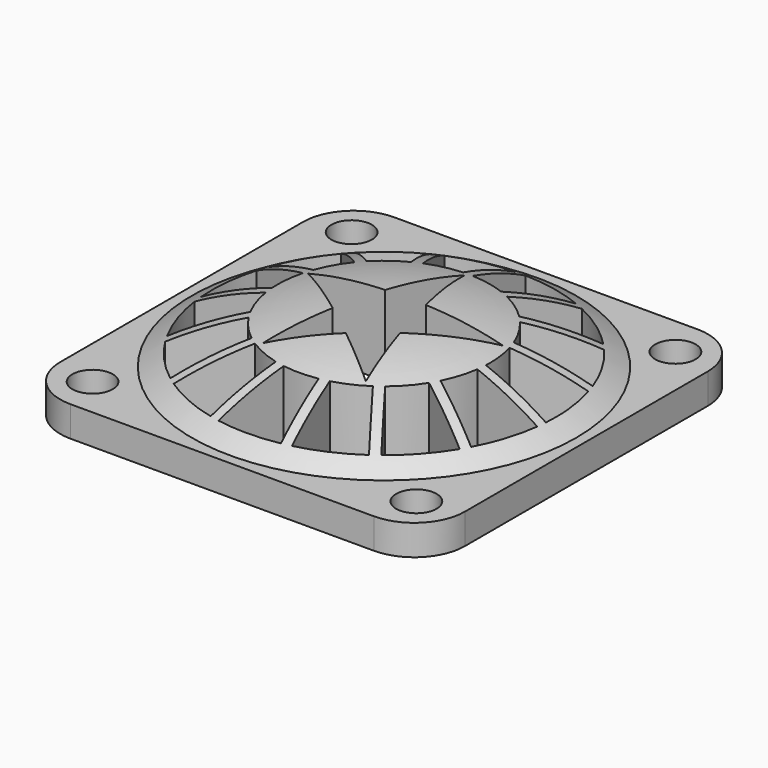
from build123d import *

# Parameters (mm, degrees)
F0_W      = 40
F0_H      = 40
F1_DEPTH  = 3
F2_R      = 2
F3_DEPTH  = 25
F4_R      = 19
F5_DEPTH  = 5
F8_DEPTH  = 25
F10_DEPTH = 25
F11_R     = 5
F12_R     = 5
F13_R     = 5
F14_R     = 5


# Not quite as in the source:
# - a fillet or chamfer that OpenCascade refuses, or shapes differently, is made with other operations: its cross-section is extruded or revolved along the edge and cut away or added


with BuildPart() as f1:
    # F0 (on Top) → F1 (new body)
    with BuildSketch(Plane.XY):
        with Locations((20, 20)):
            Rectangle(F0_W, F0_H)
    extrude(amount=F1_DEPTH)

    # F2 (on face) → F3 (cut)
    with BuildSketch(Plane.XY.offset(3)):
        with Locations((4, 36)):
            Circle(F2_R)
        with Locations((36, 36)):
            Circle(F2_R)
        with Locations((36, 4)):
            Circle(F2_R)
        with Locations((4, 4)):
            Circle(F2_R)
    extrude(amount=-F3_DEPTH, mode=Mode.SUBTRACT)

    # F4 (on face) → F5 (join)
    with BuildSketch(Plane.XY.offset(3)):
        with Locations((20, 20)):
            Circle(F4_R)
    extrude(amount=F5_DEPTH)

    # F6: fillet of radius 33 on 1 edges, made by hand

    # F6_s1 → F6_t2 (revolve, cut)
    with BuildSketch(Plane.XZ.offset(-20)):
        with BuildLine():
            ThreePointArc((39, 3), (30.6187018657, 6.7253841584), (21.5357508034, 8))
            Line((21.5357508034, 8), (21.5357508034, 8.66))
            Line((21.5357508034, 8.66), (39, 8.66))
            Line((39, 8.66), (39.66, 8))
            ThreePointArc((39.66, 8), (39.66, 5.5), (39.3492849839, 3.56))
            Line((39.3492849839, 3.56), (39, 3))
        make_face()
    revolve(axis=Axis((20, 20, 8), (0, 0, 1)), mode=Mode.SUBTRACT)

    # F7 (on face) → F8 (cut)
    with BuildSketch(Plane.XY.offset(8)):
        Polygon((22.0111904992, 22.6488580818), (20, 30), (17.9888095008, 22.6488580818), (10.3572021248, 22.6488580818), (16.6694497764, 17.8264404242), (14.9092685387, 11.3927673908), (20, 15.2819736836), (25.0907314613, 11.3927673908), (23.3305502236, 17.8264404242), (29.6427978752, 22.6488580818), align=None)
    extrude(amount=-F8_DEPTH, mode=Mode.SUBTRACT)

    # F9 (on face) → F10 (cut)
    with BuildSketch(Plane(origin=(0, 0, 0), x_dir=(1, 0, 0), z_dir=(0, 0, -1))):
        with BuildLine():
            ThreePointArc((23.7333544181, -29.8138710399), (22.0791153795, -30.2920979027), (20.3689578921, -30.4935156203))
            Line((20.3689578921, -30.4935156203), (20.3689578921, -36.995995707))
            ThreePointArc((20.3689578921, -36.995995707), (23.4306499348, -36.6502444734), (26.3796468832, -35.757541231))
            Line((26.3796468832, -35.757541231), (23.7333544181, -29.8138710399))
        make_face()
        with BuildLine():
            ThreePointArc((13.4241655667, -35.6766833707), (16.3617901212, -36.6061262454), (19.4189280081, -36.9900663724))
            Line((19.4189280081, -36.9900663724), (19.4189280081, -30.4839093539))
            ThreePointArc((19.4189280081, -30.4839093539), (17.7131930598, -30.2479516987), (16.0689624889, -29.7363722241))
            Line((16.0689624889, -29.7363722241), (13.4241655667, -35.6766833707))
        make_face()
        with BuildLine():
            Line((24.6051571238, -29.4362348352), (27.249954046, -35.3765459818))
            ThreePointArc((27.249954046, -35.3765459818), (29.9063192082, -33.8153841693), (32.2372668549, -31.8003940579))
            Line((32.2372668549, -31.8003940579), (27.4022499328, -27.446925267))
            ThreePointArc((27.4022499328, -27.446925267), (26.085539762, -28.5566468786), (24.6051571238, -29.4362348352))
        make_face()
        with BuildLine():
            ThreePointArc((30.4872159638, -19.482021885), (30.4308487622, -21.2030769299), (30.0939406684, -22.8917748499))
            Line((30.0939406684, -22.8917748499), (36.278166727, -24.9011517023))
            ThreePointArc((36.278166727, -24.9011517023), (36.895452636, -21.8824665271), (36.9577315735, -18.80194329))
            Line((36.9577315735, -18.80194329), (30.4872159638, -19.482021885))
        make_face()
        with BuildLine():
            Line((28.0450828523, -26.7473433216), (32.8773672816, -31.0983517648))
            ThreePointArc((32.8773672816, -31.0983517648), (34.6690958945, -28.5917184334), (35.9789522153, -25.802851549))
            Line((35.9789522153, -25.802851549), (29.7912291868, -23.7923384622))
            ThreePointArc((29.7912291868, -23.7923384622), (29.0397190343, -25.3416738744), (28.0450828523, -26.7473433216))
        make_face()
        with BuildLine():
            Line((30.3974644423, -18.5361922358), (36.8643232628, -17.8564979849))
            ThreePointArc((36.8643232628, -17.8564979849), (36.2004321264, -14.8477190566), (35.0043650865, -12.0081899202))
            Line((35.0043650865, -12.0081899202), (29.3698678274, -15.2612684295))
            ThreePointArc((29.3698678274, -15.2612684295), (30.0183899779, -16.8564570545), (30.3974644423, -18.5361922358))
        make_face()
        with BuildLine():
            Line((28.9031721562, -14.4337152824), (34.5344850989, -11.182475239))
            ThreePointArc((34.5344850989, -11.182475239), (32.7042097258, -8.7038477682), (30.4566075656, -6.5962931165))
            Line((30.4566075656, -6.5962931165), (26.632384421, -11.8598847126))
            ThreePointArc((26.632384421, -11.8598847126), (27.8736605522, -13.0533843126), (28.9031721562, -14.4337152824))
        make_face()
        with BuildLine():
            Line((25.8694405214, -11.2936995248), (29.6915024197, -6.033082629))
            ThreePointArc((29.6915024197, -6.033082629), (27.0113140495, -4.513183823), (24.1008076014, -3.5020190018))
            Line((24.1008076014, -3.5020190018), (22.7481014949, -9.8660008795))
            ThreePointArc((22.7481014949, -9.8660008795), (24.367503687, -10.451444531), (25.8694405214, -11.2936995248))
        make_face()
        with BuildLine():
            Line((21.8208292984, -9.6590822135), (23.1727709277, -3.2986969179))
            ThreePointArc((23.1727709277, -3.2986969179), (20.1060984783, -3.0003310881), (17.0359407482, -3.2603956812))
            Line((17.0359407482, -3.2603956812), (18.3886468546, -9.6243775589))
            ThreePointArc((18.3886468546, -9.6243775589), (20.1061657569, -9.500536736), (21.8208292984, -9.6590822135))
        make_face()
        with BuildLine():
            Line((17.4573801479, -9.8125035319), (16.1054385185, -3.4521182363))
            ThreePointArc((16.1054385185, -3.4521182363), (13.1825375163, -4.4268755453), (10.4835866672, -5.9132020218))
            Line((10.4835866672, -5.9132020218), (14.3078098118, -11.1767936179))
            ThreePointArc((14.3078098118, -11.1767936179), (15.8264708028, -10.3650815239), (17.4573801479, -9.8125035319))
        make_face()
        with BuildLine():
            Line((13.5335730688, -11.7274355401), (9.7115111705, -6.4668186443))
            ThreePointArc((9.7115111705, -6.4668186443), (7.4377777524, -8.546154698), (5.5767069054, -11.0017437073))
            Line((5.5767069054, -11.0017437073), (11.2112041645, -14.2548222166))
            ThreePointArc((11.2112041645, -14.2548222166), (12.2684169623, -12.8955912469), (13.5335730688, -11.7274355401))
        make_face()
        with BuildLine():
            Line((10.7278699518, -15.0727690973), (5.0965570091, -11.8215290539))
            ThreePointArc((5.0965570091, -11.8215290539), (3.8651403394, -14.6459077584), (3.1637455512, -17.6461656525))
            Line((3.1637455512, -17.6461656525), (9.6342611609, -18.3262442474))
            ThreePointArc((9.6342611609, -18.3262442474), (10.0472240683, -16.6545177847), (10.7278699518, -15.0727690973))
        make_face()
        with BuildLine():
            Line((9.5254023547, -19.2700656401), (3.0585435343, -18.5903713892))
            ThreePointArc((3.0585435343, -18.5903713892), (3.0823667423, -21.6714320077), (3.6619255437, -24.6975869403))
            Line((3.6619255437, -24.6975869403), (9.8496485723, -22.6870738535))
            ThreePointArc((9.8496485723, -22.6870738535), (9.5469565509, -20.9919085904), (9.5254023547, -19.2700656401))
        make_face()
        with BuildLine():
            Line((10.1340878493, -23.5935744649), (3.9498617907, -25.6029513173))
            ThreePointArc((3.9498617907, -25.6029513173), (5.2248056273, -28.4079504784), (6.9851070365, -30.9367527698))
            Line((6.9851070365, -30.9367527698), (11.8201239586, -26.5832839789))
            ThreePointArc((11.8201239586, -26.5832839789), (10.8541152088, -25.1577893895), (10.1340878493, -23.5935744649))
        make_face()
        with BuildLine():
            Line((12.4486791837, -27.2957216182), (7.6163947545, -31.6467300614))
            ThreePointArc((7.6163947545, -31.6467300614), (9.9220098478, -33.6906579276), (12.5586817592, -35.2848546882))
            Line((12.5586817592, -35.2848546882), (15.2049742243, -29.3411844972))
            ThreePointArc((15.2049742243, -29.3411844972), (13.7426804349, -28.4318415462), (12.4486791837, -27.2957216182))
        make_face()
    extrude(amount=-F10_DEPTH, mode=Mode.SUBTRACT)

    # F11
    f11_edges = [f1.edges().sort_by_distance(p)[0] for p in [
        (0, 40, 1.5),
    ]]
    fillet(f11_edges, radius=F11_R)

    # F12
    f12_edges = [f1.edges().sort_by_distance(p)[0] for p in [
        (0, 0, 1.5),
    ]]
    fillet(f12_edges, radius=F12_R)

    # F13
    f13_edges = [f1.edges().sort_by_distance(p)[0] for p in [
        (40, 0, 1.5),
    ]]
    fillet(f13_edges, radius=F13_R)

    # F14
    f14_edges = [f1.edges().sort_by_distance(p)[0] for p in [
        (40, 40, 1.5),
    ]]
    fillet(f14_edges, radius=F14_R)


solid = f1.part
